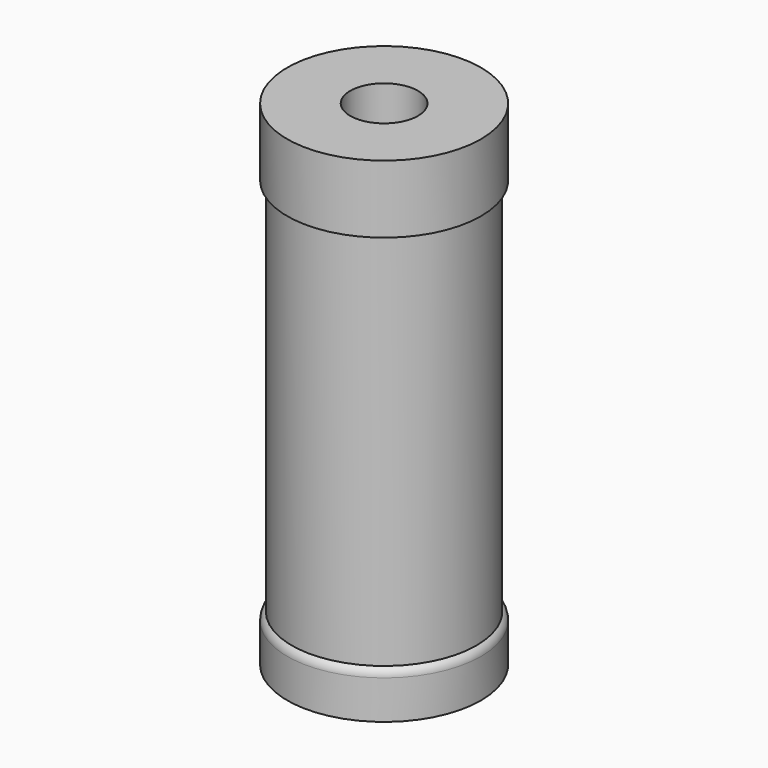
from build123d import *

# Parameters (mm, degrees)
F0_R     = 10
F0_R_2   = 9.5362250702
F0_R_3   = 4.5
F1_DEPTH = 5
F2_DEPTH = 44
F0_R_4   = 3.5
F3_DEPTH = 51
F4_R     = 10
F4_R_2   = 9.5362250702
F4_R_3   = 4.5
F5_DEPTH = 7
F6_R     = 1


with BuildPart() as f1:
    # F0 (on Top) → F1 (new body)
    with BuildSketch(Plane.XY):
        Circle(F0_R)
        Circle(F0_R_2, mode=Mode.SUBTRACT)
        Circle(F0_R_2)
        Circle(F0_R_3, mode=Mode.SUBTRACT)
    extrude(amount=F1_DEPTH)

    # F0 (on Top) → F3 (join)
    with BuildSketch(Plane.XY):
        Circle(F0_R_3)
        Circle(F0_R_4, mode=Mode.SUBTRACT)
    extrude(amount=F3_DEPTH)

    # F4 (on face) → F5 (join, through all)
    with BuildSketch(Plane.XY.offset(44)):
        Circle(F4_R)
        Circle(F4_R_2, mode=Mode.SUBTRACT)
        Circle(F4_R_2)
        Circle(F4_R_3, mode=Mode.SUBTRACT)
    extrude(amount=F5_DEPTH)

    # F6
    f6_edges = [f1.edges().sort_by_distance(p)[0] for p in [
        (-10, 0, 5),
    ]]
    fillet(f6_edges, radius=F6_R)


with BuildPart() as f2:
    # F0 (on Top) → F2 (new body)
    with BuildSketch(Plane.XY):
        Circle(F0_R_2)
        Circle(F0_R_3, mode=Mode.SUBTRACT)
    extrude(amount=F2_DEPTH)


solid = Compound([f1.part, f2.part])
